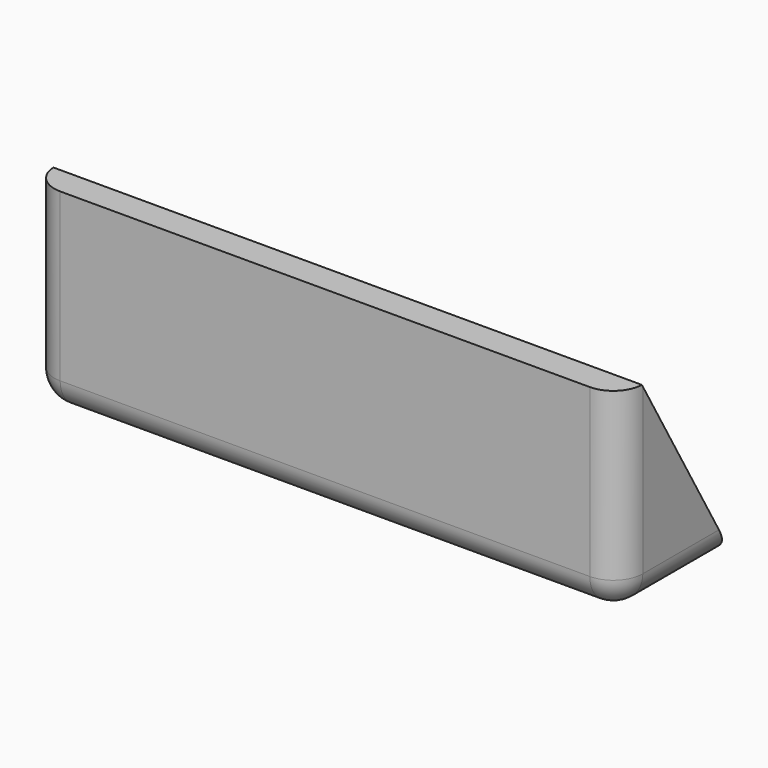
from build123d import *

# Parameters (mm, degrees)
F0_W     = 60
F0_H     = 25
F1_DEPTH = 18
F3_DEPTH = 30
F4_R     = 3


# Not quite as in the source:
# - a feature names something its author has since deleted; it is built from what else it names


with BuildPart() as f1:
    # F0 (on Front) → F1 (new body)
    with BuildSketch(Plane.XZ):
        Rectangle(F0_W, F0_H)
    extrude(amount=F1_DEPTH)

    # F2 (on Right) → F3 (cut, symmetric)
    with BuildSketch(Plane.YZ):
        Polygon((0, 12.5), (-14.4337567297, 12.5), (-11.5470053838, 7.5), (0, -12.5), (0, 0), align=None)
        Polygon((-14.4337567297, 7.5), (-14.4337567297, 12.5), (-17.3205080757, 12.5), (-19.7896268219, 12.5), (-19.7896268219, -12.5), (-17.3205080757, -12.5), (-14.4337567297, -12.5), align=None)
        Polygon((-11.5470053838, 7.5), (-14.4337567297, 12.5), (-14.4337567297, 7.5), align=None)
    extrude(amount=F3_DEPTH, both=True, mode=Mode.SUBTRACT)

    # F4
    f4_edges = [f1.edges().sort_by_distance(p)[0] for p in [
        (30, -7.216878, -12.5),
        (-30, -7.216878, -12.5),
        (0, -14.433757, -12.5),
        (30, -14.433757, -2.5),
        (-30, -14.433757, -2.5),
    ]]
    fillet(f4_edges, radius=F4_R)


solid = f1.part
